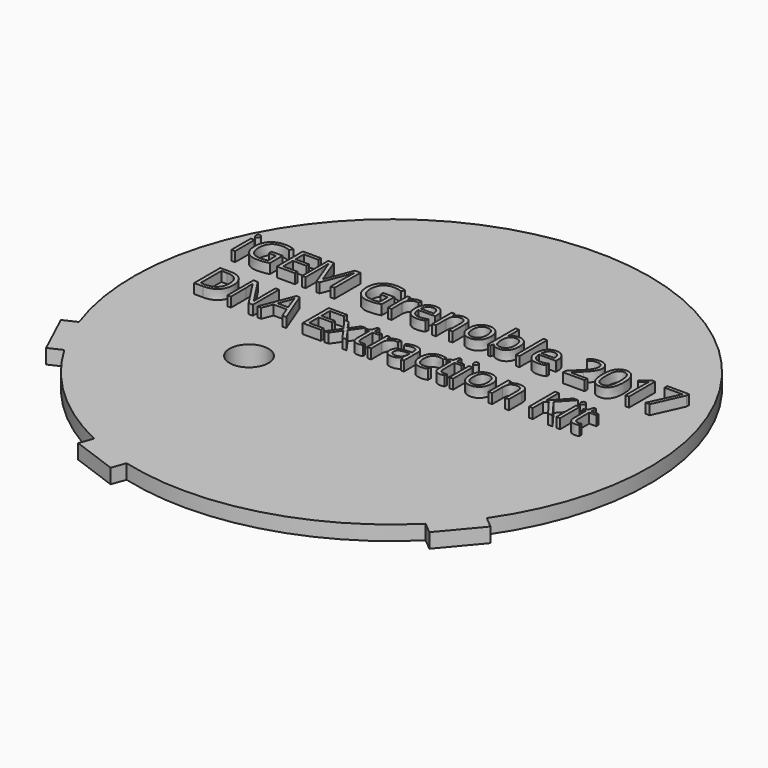
from build123d import *

# Parameters (mm, degrees)
F0_R         = 53
F1_DEPTH     = 3
F3_DEPTH     = 5
F4_R         = 4
F5_DEPTH     = 25
F6_DEPTH     = 3
F7_TEXT_SIZE = 9.3725592294
F8_DEPTH     = 2


# Not quite as in the source:
# - Text() gives the source's letters only with a copy of the font that has no kerning and outlines rounded to 1/6400 em; it was checked with that copy


with BuildPart() as f1:
    # F0 (on Top) → F1 (new body)
    with BuildSketch(Plane.XY):
        Circle(F0_R)
    extrude(amount=F1_DEPTH)

    # F2 (on face) → F3 (join)
    with BuildSketch(Plane(origin=(0, 0, 0), x_dir=(1, 0, 0), z_dir=(0, 0, -1))):
        with BuildLine():
            ThreePointArc((-5.1721314294, 7.9286940893), (-5.0792371811, 8.9281973132), (-5.0482329954, 9.9315291509))
            ThreePointArc((-5.0482329954, 9.9315291509), (-36.4216615569, 15.8766455117), (-9.3983140468, -1.134383781))
            ThreePointArc((-9.3983140468, -1.134383781), (-7.8200487667, 0.8540267468), (-6.570731456, 3.0639823976))
            ThreePointArc((-6.570731456, 3.0639823976), (-5.680852898, 5.4415470915), (-5.1721314294, 7.9286940893))
        make_face()
        with BuildLine():
            ThreePointArc((-6.570731456, 3.0639823976), (-7.8200487667, 0.8540267468), (-9.3983140468, -1.134383781))
            Line((-9.3983140468, -1.134383781), (-6.6793906857, -2.4022385663))
            Line((-6.6793906857, -2.4022385663), (-4.566299377, 2.1293003689))
            Line((-4.566299377, 2.1293003689), (-6.570731456, 3.0639823976))
        make_face()
        with BuildLine():
            Line((-2.4532080683, 6.6608393041), (-5.1721314294, 7.9286940893))
            ThreePointArc((-5.1721314294, 7.9286940893), (-5.680852898, 5.4415470915), (-6.570731456, 3.0639823976))
            Line((-6.570731456, 3.0639823976), (-4.566299377, 2.1293003689))
            Line((-4.566299377, 2.1293003689), (-2.4532080683, 6.6608393041))
        make_face()
    extrude(amount=F3_DEPTH)

    # F4 (on face) → F5 (cut)
    with BuildSketch(Plane(origin=(0, 0, -5), x_dir=(1, 0, 0), z_dir=(0, 0, -1))):
        with Locations((-21.2982329954, 9.9315291509)):
            Circle(F4_R)
    extrude(amount=-F5_DEPTH, mode=Mode.SUBTRACT)

    # F2 (on face) → F6 (join)
    with BuildSketch(Plane(origin=(0, 0, 0), x_dir=(1, 0, 0), z_dir=(0, 0, -1))):
        with BuildLine():
            ThreePointArc((-49.9331744609, 17.7673320523), (-48.0343127129, 22.3987678723), (-45.7069918435, 26.8304099227))
            Line((-45.7069918435, 26.8304099227), (-48.4259152046, 28.0982647079))
            Line((-48.4259152046, 28.0982647079), (-52.652097822, 19.0351868375))
            Line((-52.652097822, 19.0351868375), (-49.9331744609, 17.7673320523))
        make_face()
        with BuildLine():
            ThreePointArc((-22.7446852897, 47.8714872453), (-20.458700255, 48.8921423531), (-18.1270675963, 49.8037089017))
            ThreePointArc((-18.1270675963, 49.8037089017), (-15.7549896718, 50.604152996), (-13.3477590818, 51.2916886785))
            Line((-13.3477590818, 51.2916886785), (-14.3738195118, 54.1107665409))
            Line((-14.3738195118, 54.1107665409), (-23.7707457197, 50.6905651076))
            Line((-23.7707457197, 50.6905651076), (-22.7446852897, 47.8714872453))
        make_face()
        with BuildLine():
            ThreePointArc((37.2053427877, 37.7460258577), (38.9462977901, 35.9469871956), (40.6003554853, 34.0677433134))
            ThreePointArc((40.6003554853, 34.0677433134), (42.1638253258, 32.1124871957), (43.6332188846, 30.0855814265))
            Line((43.6332188846, 30.0855814265), (45.9313522139, 32.0139442555))
            Line((45.9313522139, 32.0139442555), (39.5034761171, 39.6743886867))
            Line((39.5034761171, 39.6743886867), (37.2053427877, 37.7460258577))
        make_face()
    extrude(amount=-F6_DEPTH)

    # F7 (on face) → F8 (join)
    with BuildSketch(Plane.XY.offset(3)):
        with Locations((-44.9229188291, 14.0753945401)):
            Text('iGEM Grenoble 2017', F7_TEXT_SIZE, font='Open Sans', text_align=(TextAlign.LEFT, TextAlign.BOTTOM))
        with Locations((-42.4875178919, 1.3287139882)):
            Text('DNA Extraction Kit', F7_TEXT_SIZE, font='Open Sans', text_align=(TextAlign.LEFT, TextAlign.BOTTOM))
    extrude(amount=F8_DEPTH)


solid = f1.part
